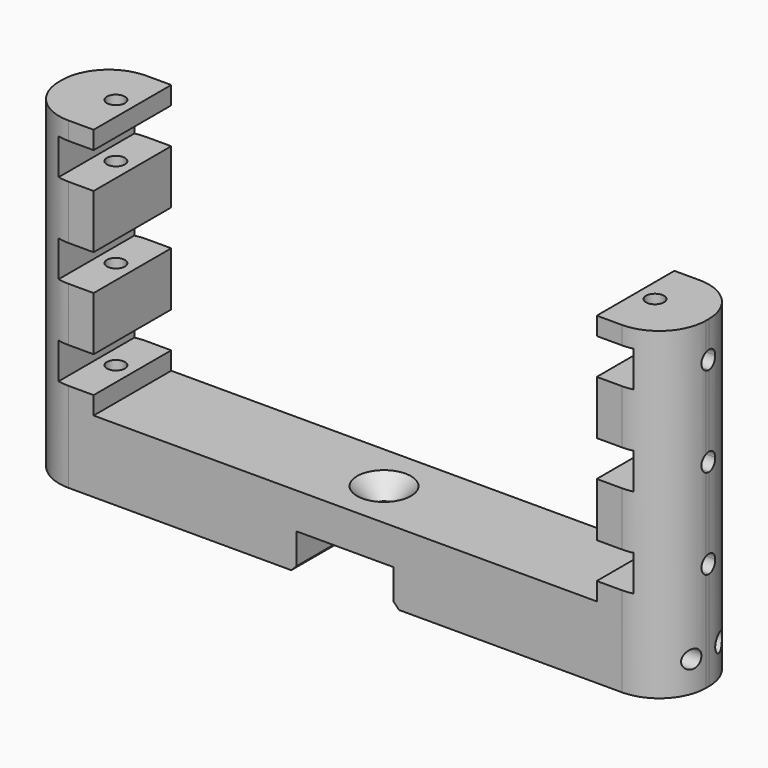
from build123d import *

# Parameters (mm, degrees)
F0_W         = 180
F0_H         = 90
F1_DEPTH     = 27
F2_W         = 140
F2_H         = 70
F3_DEPTH     = 27.001
F4_W         = 10
F4_H         = 10
F5_DEPTH     = 27.001
F6_R         = 2.5
F7_DEPTH     = 80
F9_DEPTH     = 180.001
F10_R        = 2.5
F11_DEPTH    = 20
F12_R        = 2.5
F13_DEPTH    = 20
F14_T1_DEPTH = 155
F15_W        = 27
F15_H        = 10
F16_DEPTH    = 27.0010001
F18_DEPTH    = 90.0010001
F19_SIZE     = 1.5
F20_SIZE     = 5


# Not quite as in the source:
# - a fillet or chamfer that OpenCascade refuses, or shapes differently, is made with other operations: its cross-section is extruded or revolved along the edge and cut away or added


with BuildPart() as f1:
    # F0 (on Front) → F1 (new body)
    with BuildSketch(Plane.XZ):
        with Locations((90, 45)):
            Rectangle(F0_W, F0_H)
    extrude(amount=F1_DEPTH)

    # F2 (on Front) → F3 (cut, through all)
    with BuildSketch(Plane.XZ):
        with Locations((90, 55)):
            Rectangle(F2_W, F2_H)
    extrude(amount=F3_DEPTH, mode=Mode.SUBTRACT)

    # F4 (on Front) → F5 (cut, through all)
    with BuildSketch(Plane.XZ):
        with Locations((165, 80)):
            Rectangle(F4_W, F4_H)
        with Locations((165, 55)):
            Rectangle(F4_W, F4_H)
        with Locations((165, 30)):
            Rectangle(F4_W, F4_H)
        with Locations((15, 30)):
            Rectangle(F4_W, F4_H)
        with Locations((15, 55)):
            Rectangle(F4_W, F4_H)
        with Locations((15, 80)):
            Rectangle(F4_W, F4_H)
    extrude(amount=F5_DEPTH, mode=Mode.SUBTRACT)

    # F6 (on face) → F7 (cut)
    with BuildSketch(Plane.XY.offset(90)):
        with Locations((165, -13)):
            Circle(F6_R)
        with Locations((15, -13)):
            Circle(F6_R)
    extrude(amount=-F7_DEPTH, mode=Mode.SUBTRACT)

    # F8 (on Right) → F9 (cut, through all)
    with BuildSketch(Plane.YZ):
        with BuildLine():
            Line((-13, 77.5), (-13, 82.5))
            ThreePointArc((-13, 82.5), (-15.5, 80), (-13, 77.5))
        make_face()
        with BuildLine():
            ThreePointArc((-13, 77.5), (-11.232233047, 78.232233047), (-10.5, 80))
            ThreePointArc((-10.5, 80), (-11.232233047, 81.767766953), (-13, 82.5))
            Line((-13, 82.5), (-13, 77.5))
        make_face()
        with BuildLine():
            Line((-13, 52.5), (-13, 57.5))
            ThreePointArc((-13, 57.5), (-15.5, 55), (-13, 52.5))
        make_face()
        with BuildLine():
            ThreePointArc((-10.5, 55), (-11.232233047, 56.767766953), (-13, 57.5))
            Line((-13, 57.5), (-13, 52.5))
            ThreePointArc((-13, 52.5), (-11.232233047, 53.232233047), (-10.5, 55))
        make_face()
        with BuildLine():
            Line((-13, 27.5), (-13, 32.5))
            ThreePointArc((-13, 32.5), (-15.5, 30), (-13, 27.5))
        make_face()
        with BuildLine():
            ThreePointArc((-10.5, 30), (-11.232233047, 31.767766953), (-13, 32.5))
            Line((-13, 32.5), (-13, 27.5))
            ThreePointArc((-13, 27.5), (-11.232233047, 28.232233047), (-10.5, 30))
        make_face()
    extrude(amount=F9_DEPTH, mode=Mode.SUBTRACT)

    # F10 (on Right) → F11 (cut)
    with BuildSketch(Plane.YZ):
        with Locations((-8, 8.5)):
            Circle(F10_R)
        with Locations((-18, 8.5)):
            Circle(F10_R)
    extrude(amount=F11_DEPTH, mode=Mode.SUBTRACT)

    # F12 (on face) → F13 (cut)
    with BuildSketch(Plane.YZ.offset(180)):
        with Locations((-8, 8.5)):
            Circle(F12_R)
        with Locations((-18, 8.5)):
            Circle(F12_R)
    extrude(amount=-F13_DEPTH, mode=Mode.SUBTRACT)

    # F14: fillet of radius 13 on 4 edges, made by hand

    # F14_s2 → F14_t1 (cut)
    with BuildSketch(Plane.XY.offset(-32.5)):
        with BuildLine():
            ThreePointArc((0, -13), (3.8076118446, -3.8076118446), (13, 0))
            Line((13, 0), (0, 0))
            Line((0, 0), (0, -13))
        make_face()
        with BuildLine():
            ThreePointArc((0, -14), (3.8076118446, -23.1923881554), (13, -27))
            Line((13, -27), (0, -27))
            Line((0, -27), (0, -14))
        make_face()
        with BuildLine():
            ThreePointArc((167, -27), (176.1923881554, -23.1923881554), (180, -14))
            Line((180, -14), (180, -27))
            Line((180, -27), (167, -27))
        make_face()
        with BuildLine():
            ThreePointArc((167, 0), (176.1923881554, -3.8076118446), (180, -13))
            Line((180, -13), (180, 0))
            Line((180, 0), (167, 0))
        make_face()
    extrude(amount=F14_T1_DEPTH, mode=Mode.SUBTRACT)

    # F15 (on face) → F16 (cut, through all)
    with BuildSketch(Plane.XZ.offset(27)):
        with Locations((90, 5)):
            Rectangle(F15_W, F15_H)
    extrude(amount=-F16_DEPTH, mode=Mode.SUBTRACT)

    # F17 (on Top) → F18 (cut, through all)
    with BuildSketch(Plane.XY):
        with BuildLine():
            Line((87.5, -13.5), (92.5, -13.5))
            ThreePointArc((92.5, -13.5), (90, -11), (87.5, -13.5))
        make_face()
        with BuildLine():
            ThreePointArc((87.5, -13.5), (90, -16), (92.5, -13.5))
            Line((92.5, -13.5), (87.5, -13.5))
        make_face()
    extrude(amount=F18_DEPTH, mode=Mode.SUBTRACT)

    # F19
    f19_edges = [f1.edges().sort_by_distance(p)[0] for p in [
        (76.5, -13.5, 0),
        (103.5, -13.5, 0),
    ]]
    chamfer(f19_edges, length=F19_SIZE)

    # F20
    f20_edges = [f1.edges().sort_by_distance(p)[0] for p in [
        (92.5, -13.5, 20),
    ]]
    chamfer(f20_edges, length=F20_SIZE)


solid = f1.part
